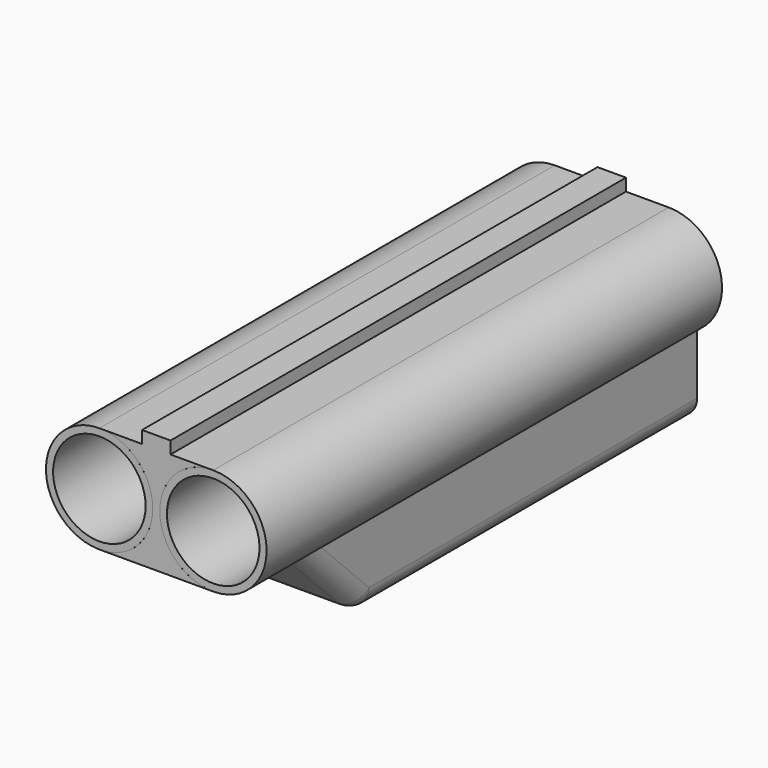
from build123d import *

# Parameters (mm, degrees)
F0_R          = 18.75
F1_DEPTH      = 200
F2_W          = 10
F2_H          = 4.3331131339
F3_DEPTH      = 200
F4_T          = -2.5
F4_2_T        = -2.5
F7_DEPTH      = 175
F8_T1_DEPTH   = 204.0142473261
F9_R          = 7
F10_R         = 4.3127157865
F11_DEPTH     = 2
F12_TEXT_SIZE = 3.3558811992
F13_DEPTH     = 1


# Not quite as in the source:
# - a fillet or chamfer that OpenCascade refuses, or shapes differently, is made with other operations: its cross-section is extruded or revolved along the edge and cut away or added
# - a feature names something its author has since deleted; it is built from what else it names
# - Text() gives the source's letters only with a copy of the font that has no kerning and outlines rounded to 1/6400 em; it was checked with that copy


with BuildPart() as f1:
    # F0 (on Front) → F1 (new body)
    with BuildSketch(Plane.XZ):
        with Locations((-20, 0)):
            Circle(F0_R)
    extrude(amount=-F1_DEPTH)

    # F4
    f4_openings = [f1.faces().sort_by_distance(p)[0] for p in [
        (-20, 0, 0),
    ]]
    offset(amount=F4_T, openings=f4_openings)


with BuildPart() as f1b:
    # F0 (on Front) → F1, piece 2 (new body)
    with BuildSketch(Plane.XZ):
        with BuildLine():
            ThreePointArc((38.75, 0), (20, 18.75), (1.25, 0))
            ThreePointArc((1.25, 0), (20, -18.75), (38.75, 0))
        make_face()
    extrude(amount=-F1_DEPTH)

    # F4#2
    f4_2_openings = [f1b.faces().sort_by_distance(p)[0] for p in [
        (20, 0, 0),
    ]]
    offset(amount=F4_2_T, openings=f4_2_openings)


with BuildPart() as f3:
    # F2 (on Front) → F3 (new body)
    with BuildSketch(Plane.XZ):
        with BuildLine():
            Line((5, 18.75), (-5, 18.75))
            Line((-5, 18.75), (-20, 18.75))
            ThreePointArc((-20, 18.75), (-1.25, 0), (-20, -18.75))
            Line((-20, -18.75), (-5, -18.75))
            Line((-5, -18.75), (5, -18.75))
            Line((5, -18.75), (20, -18.75))
            ThreePointArc((20, -18.75), (1.25, 0), (20, 18.75))
            Line((20, 18.75), (5, 18.75))
        make_face()
        with Locations((0, 20.916556567)):
            Rectangle(F2_W, F2_H)
    extrude(amount=-F3_DEPTH)


with BuildPart() as f7:
    # F6 (on offset) → F7 (new body)
    with BuildSketch(Plane.XZ.offset(-25)):
        Polygon((30, -44.014807418), (30, -19.014807418), (18.75, -19.014807418), (-18.75, -19.014807418), (-30, -19.014807418), (-30, -44.014807418), align=None)
        with BuildLine():
            Line((-30, -19.014807418), (-18.75, -19.014807418))
            ThreePointArc((-18.75, -19.014807418), (-24.6690866829, -18.0700667952), (-30, -15.3297228006))
            Line((-30, -15.3297228006), (-30, -19.014807418))
        make_face()
        with BuildLine():
            Line((18.75, -19.014807418), (30, -19.014807418))
            Line((30, -19.014807418), (30, -15.3297228006))
            ThreePointArc((30, -15.3297228006), (24.6690866829, -18.0700667952), (18.75, -19.014807418))
        make_face()
    extrude(amount=-F7_DEPTH)

    # F8: chamfer of 28 on 1 edges, made by hand

    # F8_s2 → F8_t1 (cut)
    with BuildSketch(Plane.YZ.offset(-102.007123663)):
        Polygon((53, -44.014807418), (25, -16.014807418), (25, -44.014807418), align=None)
    extrude(amount=F8_T1_DEPTH, mode=Mode.SUBTRACT)

    # F9
    f9_edges = [f7.edges().sort_by_distance(p)[0] for p in [
        (0, 53, -44.014807),
        (-30, 126.5, -44.014807),
        (-30, 39, -30.014807),
        (30, 39, -30.014807),
        (30, 126.5, -44.014807),
    ]]
    fillet(f9_edges, radius=F9_R)

    # F10 (on face) → F11 (cut)
    with BuildSketch(Plane(origin=(-30, 0, 0), x_dir=(0, -1, 0), z_dir=(-1, 0, 0))):
        with Locations((-183.5934072733, -26.5489760786)):
            Circle(F10_R)
    extrude(amount=-F11_DEPTH, mode=Mode.SUBTRACT)


with BuildPart() as f13:
    # F12 (on face) → F13 (new body)
    with BuildSketch(Plane(origin=(-30, 0, 0), x_dir=(0, -1, 0), z_dir=(-1, 0, 0))):
        with Locations((-187.0731413364, -27.6188831776)):
            Text('M&A', F12_TEXT_SIZE, font='Open Sans', font_style=FontStyle.ITALIC, text_align=(TextAlign.LEFT, TextAlign.BOTTOM))
    extrude(amount=F13_DEPTH)


solid = Compound([f1.part, f1b.part, f3.part, f7.part, f13.part])
